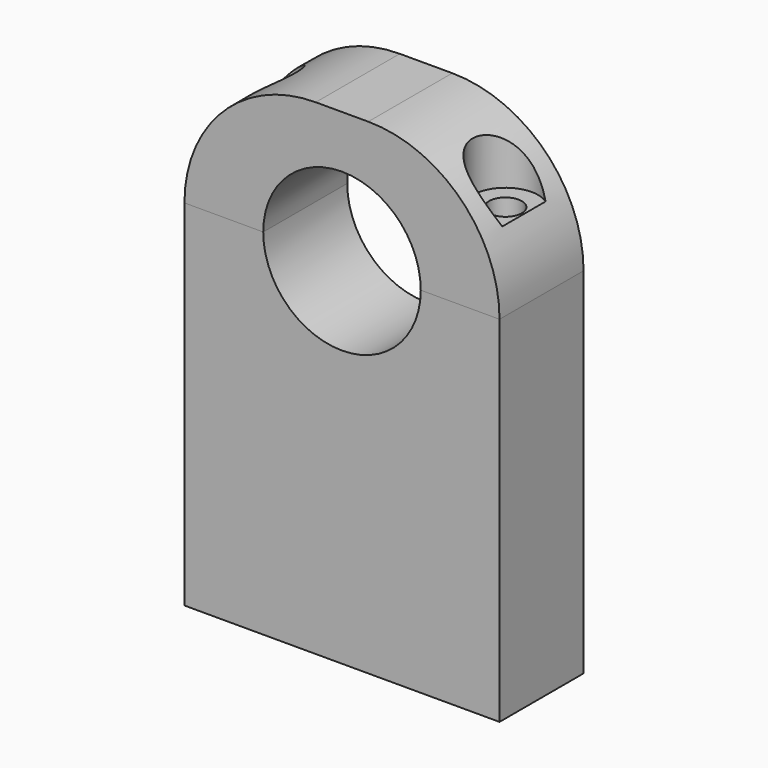
from build123d import *

# Parameters (mm, degrees)
F0_W         = 24
F0_H         = 8
F1_DEPTH     = 27
F2_W         = 24
F2_H         = 8
F3_DEPTH     = 10
F4_R         = 6
F5_DEPTH     = 12.5
F6_R         = 1.25
F7_DEPTH     = 25
F8_R         = 1.5
F9_DEPTH     = 15
F10_R        = 2.5
F11_DEPTH    = 5
F12_T1_DEPTH = 58


# Not quite as in the source:
# - a fillet or chamfer that OpenCascade refuses, or shapes differently, is made with other operations: its cross-section is extruded or revolved along the edge and cut away or added


with BuildPart() as f1:
    # F0 (on Top) → F1 (new body)
    with BuildSketch(Plane.XY):
        Rectangle(F0_W, F0_H)
    extrude(amount=-F1_DEPTH)


with BuildPart() as f3:
    # F2 (on Top) → F3 (new body)
    with BuildSketch(Plane.XY):
        Rectangle(F2_W, F2_H)
    extrude(amount=F3_DEPTH)


with BuildPart() as f5_tool:
    # F4 (on Front) → F5 (new body, symmetric)
    with BuildSketch(Plane.XZ):
        Circle(F4_R)
    extrude(amount=F5_DEPTH, both=True)


with BuildPart() as f1_1:
    add(f1.part)

    # F5: cut by f5_tool
    add(f5_tool.part, mode=Mode.SUBTRACT)


with BuildPart() as f3_1:
    add(f3.part)

    # F5: cut by f5_tool
    add(f5_tool.part, mode=Mode.SUBTRACT)


with BuildPart() as f7_tool:
    # F6 (on face) → F7 (new body)
    with BuildSketch(Plane.XY.offset(10)):
        with Locations((9.25, 0)):
            Circle(F6_R)
        with Locations((-9.25, 0)):
            Circle(F6_R)
    extrude(amount=-F7_DEPTH)


with BuildPart() as f1_2:
    add(f1_1.part)

    # F7: cut by f7_tool
    add(f7_tool.part, mode=Mode.SUBTRACT)

    # F8 (on face) → F9 (cut)
    with BuildSketch(Plane(origin=(0, 0, -27), x_dir=(1, 0, 0), z_dir=(0, 0, -1))):
        with Locations((7, 0)):
            Circle(F8_R)
        with Locations((-7, 0)):
            Circle(F8_R)
    extrude(amount=-F9_DEPTH, mode=Mode.SUBTRACT)


with BuildPart() as f3_2:
    add(f3_1.part)

    # F7: cut by f7_tool
    add(f7_tool.part, mode=Mode.SUBTRACT)

    # F10 (on face) → F11 (cut)
    with BuildSketch(Plane.XY.offset(10)):
        with Locations((9.25, 0)):
            Circle(F10_R)
        with Locations((-9.25, 0)):
            Circle(F10_R)
    extrude(amount=-F11_DEPTH, mode=Mode.SUBTRACT)

    # F12: fillet of radius 10 on 2 edges, made by hand

    # F12_s2 → F12_t1 (cut)
    with BuildSketch(Plane.XZ.offset(-29)):
        with BuildLine():
            ThreePointArc((12, 0), (9.0710678119, 7.0710678119), (2, 10))
            Line((2, 10), (12, 10))
            Line((12, 10), (12, 0))
        make_face()
        with BuildLine():
            ThreePointArc((-2, 10), (-9.0710678119, 7.0710678119), (-12, 0))
            Line((-12, 0), (-12, 10))
            Line((-12, 10), (-2, 10))
        make_face()
    extrude(amount=F12_T1_DEPTH, mode=Mode.SUBTRACT)


solid = Compound([f1_2.part, f3_2.part])
